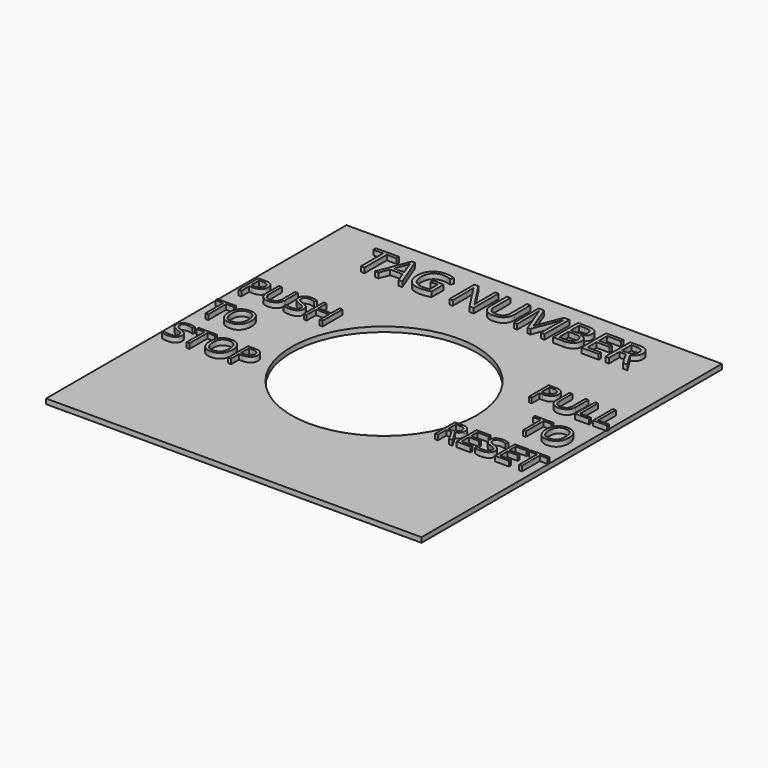
from build123d import *

# Parameters (mm, degrees)
F0_W           = 75
F0_H           = 75
F0_R           = 18.5
F1_DEPTH       = 1
F2_TEXT_SIZE   = 8.6805555556
F2_TEXT_SIZE_2 = 6.9444444444
F3_DEPTH       = 1


# Not quite as in the source:
# - Text() gives the source's letters only with a copy of the font that has no kerning and outlines rounded to 1/6400 em; it was checked with that copy


with BuildPart() as f1:
    # F0 (on Top) → F1 (new body)
    with BuildSketch(Plane.XY):
        Rectangle(F0_W, F0_H)
        Circle(F0_R, mode=Mode.SUBTRACT)
    extrude(amount=F1_DEPTH)


with BuildPart() as f3:
    # F2 (on face) → F3 (new body)
    with BuildSketch(Plane.XY.offset(1)):
        with Locations((-27.9018825955, 26.5704803169)):
            Text('TAG NUMBER', F2_TEXT_SIZE, font='Open Sans', text_align=(TextAlign.LEFT, TextAlign.BOTTOM))
        with Locations((-36.5045923716, 8.4374530986)):
            Text('PUSH', F2_TEXT_SIZE_2, font='Open Sans', text_align=(TextAlign.LEFT, TextAlign.BOTTOM))
        with Locations((-36.5045923716, -1.0069913458)):
            Text('TO', F2_TEXT_SIZE_2, font='Open Sans', text_align=(TextAlign.LEFT, TextAlign.BOTTOM))
        with Locations((-36.5045923716, -10.4514357903)):
            Text('STOP', F2_TEXT_SIZE_2, font='Open Sans', text_align=(TextAlign.LEFT, TextAlign.BOTTOM))
        with Locations((21.4284209662, 8.5318651795)):
            Text('PULL', F2_TEXT_SIZE_2, font='Open Sans', text_align=(TextAlign.LEFT, TextAlign.BOTTOM))
        with Locations((26.8418324246, -0.9125792649)):
            Text('TO', F2_TEXT_SIZE_2, font='Open Sans', text_align=(TextAlign.LEFT, TextAlign.BOTTOM))
        with Locations((17.819479994, -10.3570237094)):
            Text('RESET', F2_TEXT_SIZE_2, font='Open Sans', text_align=(TextAlign.LEFT, TextAlign.BOTTOM))
    extrude(amount=F3_DEPTH)


solid = Compound([f1.part, f3.part])
